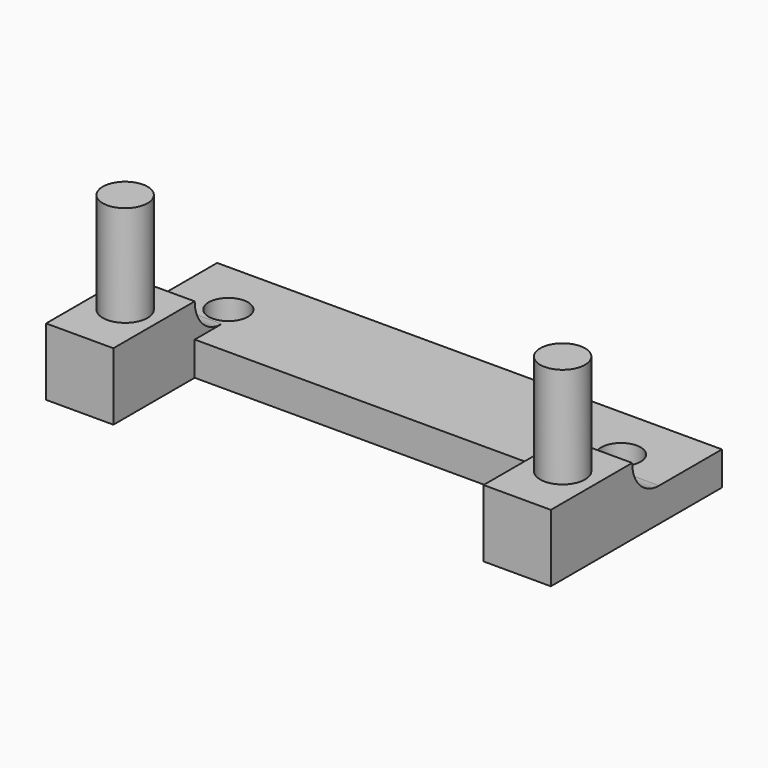
from build123d import *

# Parameters (mm, degrees)
F0_W     = 6
F0_H     = 9.0617471188
F0_R     = 2
F1_DEPTH = 3
F2_D     = 3.5
F3_DEPTH = 15
F4_DEPTH = 6
F5_R     = 2.99999


# Not quite as in the source:
# - a fillet or chamfer is up to 0.001 mm smaller than in the source, because OpenCascade refuses the exact size
# - a feature names something its author has since deleted; it is built from what else it names


with BuildPart() as f1:
    # F0 (on Top) → F1 (new body)
    with BuildSketch(Plane.XY):
        Polygon((22.5, 5), (-22.5, 5), (-22.5, -5), (-16.5, -5), (16.5, -5), (22.5, -5), align=None)
        with Locations((-19.5, -9.5308735594)):
            Rectangle(F0_W, F0_H)
        with Locations((-19.5, -9)):
            Circle(F0_R, mode=Mode.SUBTRACT)
        with Locations((19.5, -9.5308735594)):
            Rectangle(F0_W, F0_H)
        with Locations((19.5, -9)):
            Circle(F0_R, mode=Mode.SUBTRACT)
        with Locations((-19.5, -9)):
            Circle(F0_R)
        with Locations((19.5, -9)):
            Circle(F0_R)
    extrude(amount=F1_DEPTH)

    # F2 (through all)
    with Locations(Plane(origin=(0, 0, 0), x_dir=(1, 0, 0), z_dir=(0, 0, -1))):
        with Locations((-17.5, 0), (17.5, 0)):
            Hole(F2_D / 2)

    # F0 (on Top) → F3 (join)
    with BuildSketch(Plane.XY):
        with Locations((-19.5, -9)):
            Circle(F0_R)
        with Locations((19.5, -9)):
            Circle(F0_R)
    extrude(amount=F3_DEPTH)

    # F0 (on Top) → F4 (join)
    with BuildSketch(Plane.XY):
        with Locations((-19.5, -9.5308735594)):
            Rectangle(F0_W, F0_H)
        with Locations((-19.5, -9)):
            Circle(F0_R, mode=Mode.SUBTRACT)
        with Locations((19.5, -9.5308735594)):
            Rectangle(F0_W, F0_H)
        with Locations((19.5, -9)):
            Circle(F0_R, mode=Mode.SUBTRACT)
        with Locations((-19.5, -9)):
            Circle(F0_R)
    extrude(amount=F4_DEPTH)

    # F5 (radius 3 in the source; OpenCascade refuses exactly that, so slightly less here)
    f5_edges = [f1.edges().sort_by_distance(p)[0] for p in [
        (-19.5, -5, 3),
        (19.5, -5, 3),
    ]]
    fillet(f5_edges, radius=F5_R)


solid = f1.part
